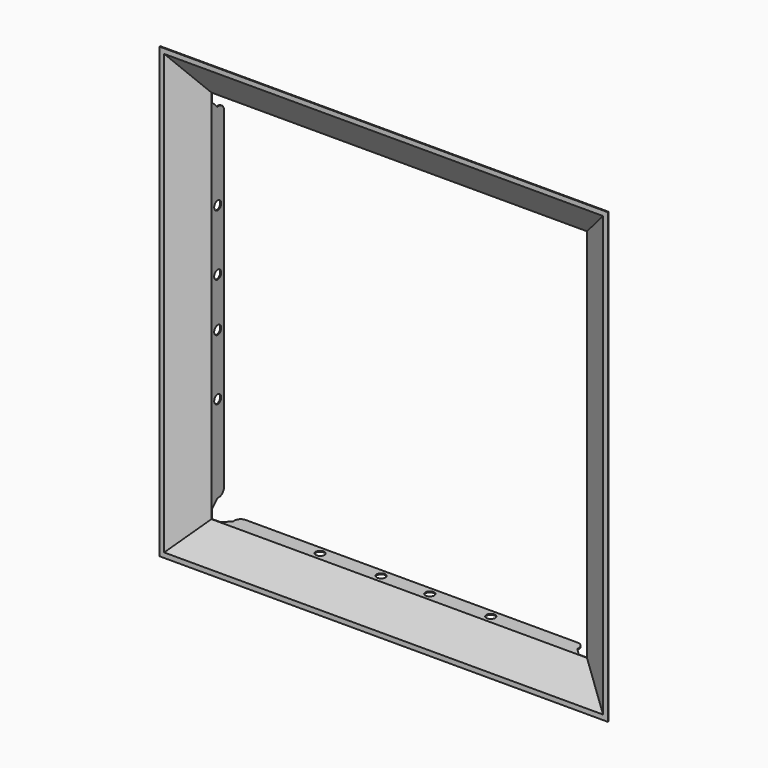
from build123d import *

# Parameters (mm, degrees)
F0_W             = 450
F0_H             = 450
F2_W             = 385
F2_H             = 385
F5_W             = 385
F5_H             = 385
F3_FACE_W        = 385
F3_FACE_H        = 385
F7_T             = 1
F12_COPIES_COUNT = 2
F12_COPIES_ANGLE = 90
F14_R            = 4.5
F15_DEPTH        = 420.4090421903
F16_R            = 4.5
F17_DEPTH        = 420.4090421903
F18_W            = 1
F18_H            = 5


# Not quite as in the source:
# - a feature of the source that left no trace in its solid (it failed there, or was rolled back) is left out
# - a pattern or mirror of a feature is missing from the dataset's text; its kind, count and spacing are read off the source's solid


with BuildPart() as f3:
    # F0 (on Front) → F3 section 0
    with BuildSketch(Plane.XZ):
        Rectangle(F0_W, F0_H)
    # F2 (on offset) → F3 section 1
    with BuildSketch(Plane.XZ.offset(-20)):
        Rectangle(F2_W, F2_H)
    loft()

    # F5 (on offset) → F6 section 0
    with BuildSketch(Plane.XZ.offset(-36)):
        Rectangle(F5_W, F5_H)
    # F3_face (on face) → F6 section 1
    with BuildSketch(Plane(origin=(0, 20, 0), x_dir=(-1, 0, 0), z_dir=(0, 1, 0))):
        Rectangle(F3_FACE_W, F3_FACE_H)
    loft()

    # F7
    f7_openings = [f3.faces().sort_by_distance(p)[0] for p in [
        (0, 0, 0),
        (0, 36, 0),
    ]]
    offset(amount=F7_T, openings=f7_openings, kind=Kind.INTERSECTION)

    # F8 (on face) → F10 (revolve, cut)
    with BuildSketch(Plane(origin=(-193.5, 0, 0), x_dir=(0, -1, 0), z_dir=(-1, 0, 0))):
        with BuildLine():
            Line((-20.558795194, -193.5), (-20.558795194, -192.5))
            add(Edge.make_bspline(
                [(-36, -192.5), (-20.558795194, -192.5)],
                knots=[0, 0, 0.9650753004, 0.9650753004], degree=1))
            Line((-36, -192.5), (-36, -193.5))
            Line((-36, -193.5), (-20.558795194, -193.5))
        make_face()
    revolve(axis=Axis((-193.5, 28.279397597, -193.5), (0, 1, 0)), mode=Mode.SUBTRACT)

    # F11 (on face) → F12 (revolve, cut)
    with BuildSketch(Plane.YZ.offset(193.5)):
        with BuildLine():
            Line((27.6298630059, -176.4289321881), (20.558795194, -183.5))
            Line((20.558795194, -183.5), (20.558795194, -192.5))
            add(Edge.make_bspline(
                [(36, -192.5), (20.558795194, -192.5)],
                knots=[0, 0, 0.9650753004, 0.9650753004], degree=1))
            Line((36, -192.5), (36, -170.9152411143))
            ThreePointArc((36, -170.9152411143), (33.0658481949, -175.5710584905), (27.6298630059, -176.4289321881))
        make_face()
        with BuildLine():
            add(Edge.make_bspline(
                [(36, -192.5), (20.558795194, -192.5)],
                knots=[0, 0, 0.9650753004, 0.9650753004], degree=1))
            Line((20.558795194, -192.5), (20.558795194, -193.5))
            Line((20.558795194, -193.5), (36, -193.5))
            Line((36, -193.5), (36, -192.5))
        make_face()
    f12 = revolve(axis=Axis((193.5, 28.279397597, -193.5), (0, 1, 0)), mode=Mode.SUBTRACT)

    # F12_copies: F12 ×2 about axis
    f12_copies_axis = Axis((1e-06, 0, -2.1e-05), (0, 1, 0))
    for i in range(1, F12_COPIES_COUNT):
        add(f12.rotate(f12_copies_axis, i * F12_COPIES_ANGLE / (F12_COPIES_COUNT - 1)), mode=Mode.SUBTRACT)

    # F12_copies1: F12 across plane
    add(f12.mirror(Plane(origin=(0, 0, 0), x_dir=(0.7071067823, 0, 0.7071067801), z_dir=(-0.7071067801, -6e-10, 0.7071067823))), mode=Mode.SUBTRACT)

    # F11 (on face) → F13 (revolve, cut)
    with BuildSketch(Plane.YZ.offset(193.5)):
        with BuildLine():
            Line((20.558795194, 193.5), (20.558795194, 192.5))
            add(Edge.make_bspline(
                [(36, 192.5), (20.558795194, 192.5)],
                knots=[0, 0, 0.9650753004, 0.9650753004], degree=1))
            Line((36, 192.5), (36, 193.5))
            Line((36, 193.5), (20.558795194, 193.5))
        make_face()
        with BuildLine():
            add(Edge.make_bspline(
                [(36, 192.5), (20.558795194, 192.5)],
                knots=[0, 0, 0.9650753004, 0.9650753004], degree=1))
            Line((20.558795194, 192.5), (20.558795194, 183.5))
            Line((20.558795194, 183.5), (27.6298630059, 176.4289321881))
            ThreePointArc((27.6298630059, 176.4289321881), (33.0658481949, 175.5710584905), (36, 170.9152411143))
            Line((36, 170.9152411143), (36, 192.5))
        make_face()
    revolve(axis=Axis((193.5, 28.279397597, 193.5), (0, 1, 0)), mode=Mode.SUBTRACT)

    # F14 (on face) → F15 (cut, through all)
    with BuildSketch(Plane(origin=(0, 0, -193.5), x_dir=(1, 0, 0), z_dir=(0, 0, -1))):
        with Locations((-25, -28)):
            Circle(F14_R)
        with Locations((25, -28)):
            Circle(F14_R)
        with Locations((-87.5, -28)):
            Circle(F14_R)
        with Locations((87.5, -28)):
            Circle(F14_R)
    extrude(amount=-F15_DEPTH, mode=Mode.SUBTRACT)

    # F16 (on face) → F17 (cut, through all)
    with BuildSketch(Plane(origin=(-193.5, 0, 0), x_dir=(0, -1, 0), z_dir=(-1, 0, 0))):
        with Locations((-28, 25)):
            Circle(F16_R)
        with Locations((-28, 87.5)):
            Circle(F16_R)
        with Locations((-28, -25)):
            Circle(F16_R)
        with Locations((-28, -87.5)):
            Circle(F16_R)
    extrude(amount=-F17_DEPTH, mode=Mode.SUBTRACT)

    # F19: sweep along a path in F19_path
    with BuildLine(Plane(origin=(-225, 0, 225), x_dir=(0, 0, -1), z_dir=(0, 1, 0))) as f19_path:
        Line((0, 0), (450, 0))
        Line((450, 0), (450, -450))
        Line((450, -450), (0, -450))
        Line((0, -450), (0, 0))
    # F18 (on Right) → F19 (sweep)
    with BuildSketch(Plane.YZ):
        with Locations((0.5, 227.5)):
            Rectangle(F18_W, F18_H)
    sweep(path=f19_path.line, transition=Transition.RIGHT)


solid = f3.part
